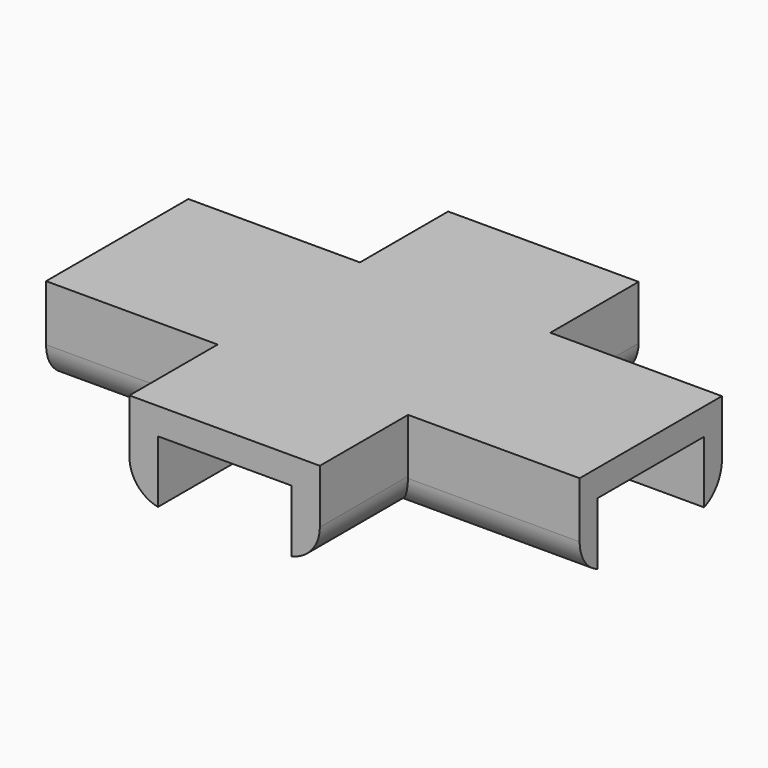
from build123d import *

# Parameters (mm, degrees)
F2_DEPTH     = 5
F3_DEPTH     = 3.5
F4_T1_DEPTH  = 14.2822071908
F4_T3_DEPTH  = 11.1004623397
F4_T5_DEPTH  = 14.2822071908
F4_T7_DEPTH  = 11.1004623397
F4_T13_DEPTH = 11.1004623397
F4_T18_DEPTH = 14.2822071908
F4_T26_DEPTH = 14.2822071908
F4_T31_DEPTH = 11.1004623397
F4_T39_DEPTH = 14.2822071908
F4_T44_DEPTH = 11.1004623397
F4_T52_DEPTH = 11.1004623397
F4_T57_DEPTH = 14.2822071908


# Not quite as in the source:
# - a fillet or chamfer that OpenCascade refuses, or shapes differently, is made with other operations: its cross-section is extruded or revolved along the edge and cut away or added


with BuildPart() as f2:
    # F1 (on Top) → F2 (new body)
    with BuildSketch(Plane.XY):
        Polygon((-5.3529168636, -11.2), (5.3529168636, -11.2), (5.3529168636, -5), (15, -5), (15, 5), (5.3529168636, 5), (5.3529168636, 11.2), (-5.3529168636, 11.2), (-5.3529168636, 5), (-15, 5), (-15, -5), (-5.3529168636, -5), align=None)
    extrude(amount=F2_DEPTH)

    # F0 (on Top) → F3 (cut)
    with BuildSketch(Plane.XY):
        Polygon((-3.75, -11.2), (3.75, -11.2), (3.75, -3.75), (15, -3.75), (15, 3.75), (3.75, 3.75), (3.75, 11.2), (-3.75, 11.2), (-3.75, 3.75), (-15, 3.75), (-15, -3.75), (-3.75, -3.75), align=None)
    extrude(amount=F3_DEPTH, mode=Mode.SUBTRACT)

    # F4: fillet of radius 2 on 8 edges, made by hand

    # F4_s2 → F4_t1 (cut)
    with BuildSketch(Plane.YZ.offset(5.3529168636)):
        with BuildLine():
            ThreePointArc((5, 1.8540496218), (4.6583123952, 0.736015633), (3.75, 0))
            Line((3.75, 0), (5, 0))
            Line((5, 0), (5, 1.8540496218))
        make_face()
        with BuildLine():
            ThreePointArc((-5, 1.8540496218), (-4.6583123952, 0.736015633), (-3.75, 0))
            Line((-3.75, 0), (-5, 0))
            Line((-5, 0), (-5, 1.8540496218))
        make_face()
    extrude(amount=F4_T1_DEPTH, mode=Mode.SUBTRACT)

    # F4_s4 → F4_t3 (cut)
    with BuildSketch(Plane.XZ.offset(-16.1004623397)):
        with BuildLine():
            ThreePointArc((-3.75, 0), (-4.9011685022, 0.6941214052), (-5.3529168636, 1.9601849359))
            Line((-5.3529168636, 1.9601849359), (-5.3529168636, 0))
            Line((-5.3529168636, 0), (-3.75, 0))
        make_face()
        with BuildLine():
            ThreePointArc((5.3529168636, 1.9601849359), (4.9011685022, 0.6941214052), (3.75, 0))
            Line((3.75, 0), (5.3529168636, 0))
            Line((5.3529168636, 0), (5.3529168636, 1.9601849359))
        make_face()
    extrude(amount=F4_T3_DEPTH, mode=Mode.SUBTRACT)

    # F4_s6 → F4_t5 (cut)
    with BuildSketch(Plane.YZ.offset(-19.6351240544)):
        with BuildLine():
            ThreePointArc((3.75, 0), (4.6583123952, 0.736015633), (5, 1.8540496218))
            Line((5, 1.8540496218), (5, 0))
            Line((5, 0), (3.75, 0))
        make_face()
        with BuildLine():
            ThreePointArc((-5, 1.8540496218), (-4.6583123952, 0.736015633), (-3.75, 0))
            Line((-3.75, 0), (-5, 0))
            Line((-5, 0), (-5, 1.8540496218))
        make_face()
    extrude(amount=F4_T5_DEPTH, mode=Mode.SUBTRACT)

    # F4_s8 → F4_t7 (cut)
    with BuildSketch(Plane.XZ.offset(5)):
        with BuildLine():
            ThreePointArc((-5.3529168636, 1.9601849359), (-4.9011685022, 0.6941214052), (-3.75, 0))
            Line((-3.75, 0), (-5.3529168636, 0))
            Line((-5.3529168636, 0), (-5.3529168636, 1.9601849359))
        make_face()
        with BuildLine():
            ThreePointArc((5.3529168636, 1.9601849359), (4.9011685022, 0.6941214052), (3.75, 0))
            Line((3.75, 0), (5.3529168636, 0))
            Line((5.3529168636, 0), (5.3529168636, 1.9601849359))
        make_face()
    extrude(amount=F4_T7_DEPTH, mode=Mode.SUBTRACT)


with BuildPart() as f4_tool11:
    # F4_s12 → F4_t13 (new body)
    with BuildSketch(Plane.XZ.offset(-0.0995376603)):
        with BuildLine():
            ThreePointArc((5.3529168636, 1.9601849359), (4.9011685022, 0.6941214052), (3.75, 0))
            Line((3.75, 0), (5.3529168636, 0))
            Line((5.3529168636, 0), (5.3529168636, 1.9601849359))
        make_face()
    extrude(amount=-F4_T13_DEPTH)

    split(bisect_by=Plane.XZ.offset(-5), keep=Keep.TOP)

    split(bisect_by=Plane.XZ.offset(-3.75), keep=Keep.BOTTOM)


with BuildPart() as f4_tool16:
    # F4_s17 → F4_t18 (new body)
    with BuildSketch(Plane.YZ.offset(15)):
        with BuildLine():
            ThreePointArc((5, 1.8540496218), (4.6583123952, 0.736015633), (3.75, 0))
            Line((3.75, 0), (5, 0))
            Line((5, 0), (5, 1.8540496218))
        make_face()
    extrude(amount=-F4_T18_DEPTH)

    split(bisect_by=Plane.YZ.offset(5.3529168636), keep=Keep.BOTTOM)

    split(bisect_by=Plane.YZ.offset(3.75), keep=Keep.TOP)


with BuildPart() as f4_tool11_1:
    add(f4_tool11.part)

    # F4_t21: intersect F4_tool16
    add(f4_tool16.part, mode=Mode.INTERSECT)


with BuildPart() as f2_1:
    add(f2.part)

    # F4_t9: cut F4_tool11
    add(f4_tool11_1.part, mode=Mode.SUBTRACT)


with BuildPart() as f4_tool24:
    # F4_s25 → F4_t26 (new body)
    with BuildSketch(Plane.YZ.offset(-0.7177928092)):
        with BuildLine():
            ThreePointArc((3.75, 0), (4.6583123952, 0.736015633), (5, 1.8540496218))
            Line((5, 1.8540496218), (5, 0))
            Line((5, 0), (3.75, 0))
        make_face()
    extrude(amount=-F4_T26_DEPTH)

    split(bisect_by=Plane.YZ.offset(-3.75), keep=Keep.BOTTOM)

    split(bisect_by=Plane.YZ.offset(-5.3529168636), keep=Keep.TOP)


with BuildPart() as f4_tool29:
    # F4_s30 → F4_t31 (new body)
    with BuildSketch(Plane.XZ.offset(-11.2)):
        with BuildLine():
            ThreePointArc((-3.75, 0), (-4.9011685022, 0.6941214052), (-5.3529168636, 1.9601849359))
            Line((-5.3529168636, 1.9601849359), (-5.3529168636, 0))
            Line((-5.3529168636, 0), (-3.75, 0))
        make_face()
    extrude(amount=F4_T31_DEPTH)

    split(bisect_by=Plane.XZ.offset(-5), keep=Keep.TOP)

    split(bisect_by=Plane.XZ.offset(-3.75), keep=Keep.BOTTOM)


with BuildPart() as f4_tool24_1:
    add(f4_tool24.part)

    # F4_t34: intersect F4_tool29
    add(f4_tool29.part, mode=Mode.INTERSECT)


with BuildPart() as f2_2:
    add(f2_1.part)

    # F4_t22: cut F4_tool24
    add(f4_tool24_1.part, mode=Mode.SUBTRACT)


with BuildPart() as f4_tool37:
    # F4_s38 → F4_t39 (new body)
    with BuildSketch(Plane.YZ.offset(-15)):
        with BuildLine():
            ThreePointArc((-5, 1.8540496218), (-4.6583123952, 0.736015633), (-3.75, 0))
            Line((-3.75, 0), (-5, 0))
            Line((-5, 0), (-5, 1.8540496218))
        make_face()
    extrude(amount=F4_T39_DEPTH)

    split(bisect_by=Plane.YZ.offset(-5.3529168636), keep=Keep.TOP)

    split(bisect_by=Plane.YZ.offset(-3.75), keep=Keep.BOTTOM)


with BuildPart() as f4_tool42:
    # F4_s43 → F4_t44 (new body)
    with BuildSketch(Plane.XZ.offset(0.0995376603)):
        with BuildLine():
            ThreePointArc((-5.3529168636, 1.9601849359), (-4.9011685022, 0.6941214052), (-3.75, 0))
            Line((-3.75, 0), (-5.3529168636, 0))
            Line((-5.3529168636, 0), (-5.3529168636, 1.9601849359))
        make_face()
    extrude(amount=F4_T44_DEPTH)

    split(bisect_by=Plane.XZ.offset(5), keep=Keep.BOTTOM)

    split(bisect_by=Plane.XZ.offset(3.75), keep=Keep.TOP)


with BuildPart() as f4_tool37_1:
    add(f4_tool37.part)

    # F4_t47: intersect F4_tool42
    add(f4_tool42.part, mode=Mode.INTERSECT)


with BuildPart() as f2_3:
    add(f2_2.part)

    # F4_t35: cut F4_tool37
    add(f4_tool37_1.part, mode=Mode.SUBTRACT)


with BuildPart() as f4_tool50:
    # F4_s51 → F4_t52 (new body)
    with BuildSketch(Plane.XZ.offset(11.2)):
        with BuildLine():
            ThreePointArc((5.3529168636, 1.9601849359), (4.9011685022, 0.6941214052), (3.75, 0))
            Line((3.75, 0), (5.3529168636, 0))
            Line((5.3529168636, 0), (5.3529168636, 1.9601849359))
        make_face()
    extrude(amount=-F4_T52_DEPTH)

    split(bisect_by=Plane.XZ.offset(5), keep=Keep.BOTTOM)

    split(bisect_by=Plane.XZ.offset(3.75), keep=Keep.TOP)


with BuildPart() as f4_tool55:
    # F4_s56 → F4_t57 (new body)
    with BuildSketch(Plane.YZ.offset(0.7177928092)):
        with BuildLine():
            ThreePointArc((-5, 1.8540496218), (-4.6583123952, 0.736015633), (-3.75, 0))
            Line((-3.75, 0), (-5, 0))
            Line((-5, 0), (-5, 1.8540496218))
        make_face()
    extrude(amount=F4_T57_DEPTH)

    split(bisect_by=Plane.YZ.offset(5.3529168636), keep=Keep.BOTTOM)

    split(bisect_by=Plane.YZ.offset(3.75), keep=Keep.TOP)


with BuildPart() as f4_tool50_1:
    add(f4_tool50.part)

    # F4_t60: intersect F4_tool55
    add(f4_tool55.part, mode=Mode.INTERSECT)


with BuildPart() as f2_4:
    add(f2_3.part)

    # F4_t48: cut F4_tool50
    add(f4_tool50_1.part, mode=Mode.SUBTRACT)


solid = f2_4.part
